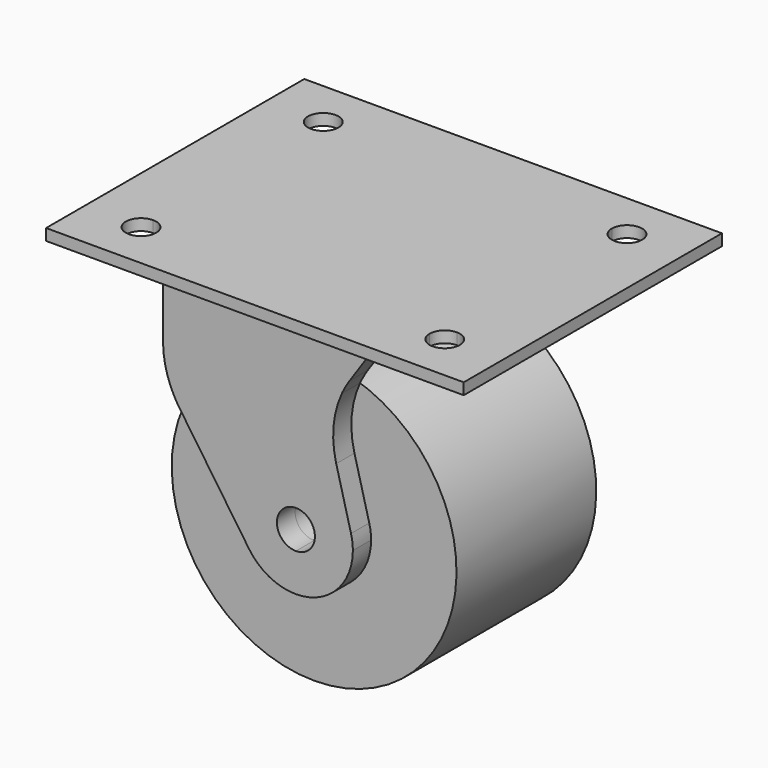
from build123d import *

# Parameters (mm, degrees)
F1_DEPTH = 23
F2_W     = 110
F2_H     = 85
F3_DEPTH = 3
F5_DEPTH = 6
F6_W     = 34.7799539885
F6_H     = 6
F7_DEPTH = 1
F8_DEPTH = 1


with BuildPart() as f1:
    # F0 (on Front) → F1 (new body, symmetric)
    with BuildSketch(Plane.XZ):
        with BuildLine():
            ThreePointArc((37.5, -57.5), (-26.5165042945, -30.9834957055), (0, -95))
            ThreePointArc((0, -95), (26.5165042945, -84.0165042945), (37.5, -57.5))
        make_face()
        with BuildLine():
            ThreePointArc((5, -57.5), (3.5355339059, -61.0355339059), (0, -62.5))
            ThreePointArc((0, -62.5), (-3.5355339059, -53.9644660941), (5, -57.5))
        make_face(mode=Mode.SUBTRACT)
    extrude(amount=F1_DEPTH, both=True)


with BuildPart() as f3:
    # F2 (on Top) → F3 (new body)
    with BuildSketch(Plane.XY):
        Rectangle(F2_W, F2_H)
        with BuildLine():
            Line((36, -30), (-36, -30))
            ThreePointArc((-36, -30), (-42.8284271247, -32.8284271247), (-40, -26))
            Line((-40, -26), (-40, 26))
            ThreePointArc((-40, 26), (-42.8284271247, 32.8284271247), (-36, 30))
            Line((-36, 30), (36, 30))
            ThreePointArc((36, 30), (40, 34), (44, 30))
            ThreePointArc((44, 30), (42.8284271247, 27.1715728753), (40, 26))
            Line((40, 26), (40, -26))
            ThreePointArc((40, -26), (42.8284271247, -27.1715728753), (44, -30))
            ThreePointArc((44, -30), (40, -34), (36, -30))
        make_face(mode=Mode.SUBTRACT)
        with BuildLine():
            ThreePointArc((-40, -26), (-37.1715728753, -27.1715728753), (-36, -30))
            Line((-36, -30), (36, -30))
            ThreePointArc((36, -30), (37.1715728753, -27.1715728753), (40, -26))
            Line((40, -26), (40, 26))
            ThreePointArc((40, 26), (37.1715728753, 27.1715728753), (36, 30))
            Line((36, 30), (-36, 30))
            ThreePointArc((-36, 30), (-37.1715728753, 27.1715728753), (-40, 26))
            Line((-40, 26), (-40, -26))
        make_face()
    extrude(amount=-F3_DEPTH)

    # F6 (on face) → F7 (cut)
    with BuildSketch(Plane(origin=(0, 0, -3), x_dir=(1, 0, 0), z_dir=(0, 0, -1))):
        Polygon((24.8050460115, -22.5), (0, -22.5), (0, -28.5), (24.8050460115, -28.6190058787), align=None)
        with Locations((-17.3899769943, -25.5)):
            Rectangle(F6_W, F6_H)
        Polygon((0, 22.5), (24.8050460115, 22.5), (24.8050460115, 28.6190058787), (0, 28.5), (-34.7799539885, 28.5), (-34.7799539885, 22.5), align=None)
    extrude(amount=-F7_DEPTH, mode=Mode.SUBTRACT)


with BuildPart() as f5:
    # F4 (on face) → F5 (new body)
    with BuildSketch(Plane.XZ.offset(23)):
        with BuildLine():
            ThreePointArc((-31.7587456306, -37.5592859714), (-12.5289492083, -22.1549093687), (12.1096103032, -22.0090527274))
            ThreePointArc((12.1096103032, -22.0090527274), (13.0382727302, -20.194540616), (14.1116697761, -18.4617143444))
            Line((14.1116697761, -18.4617143444), (24.5849639177, -3))
            Line((24.5849639177, -3), (0, -3))
            Line((0, -3), (-35, -3))
            Line((-35, -3), (-35, -25.248437561))
            ThreePointArc((-35, -25.248437561), (-34.1761105305, -31.6136303796), (-31.7587456306, -37.5592859714))
        make_face()
        with BuildLine():
            ThreePointArc((-12.3687979141, -65.9860378364), (-6.2301711882, -43.8550387701), (14.5137450016, -53.7117014336))
            Line((14.5137450016, -53.7117014336), (10.6205409153, -38.7960419739))
            ThreePointArc((10.6205409153, -38.7960419739), (9.9078937869, -30.273289816), (12.1096103032, -22.0090527274))
            ThreePointArc((12.1096103032, -22.0090527274), (-12.5289492083, -22.1549093687), (-31.7587456306, -37.5592859714))
            ThreePointArc((-31.7587456306, -37.5592859714), (-31.2065084773, -38.4879238879), (-30.6146631901, -39.3918339551))
            Line((-30.6146631901, -39.3918339551), (-12.3687979141, -65.9860378364))
        make_face()
        with BuildLine():
            ThreePointArc((-12.3687979141, -65.9860378364), (4.4422984641, -71.8271066289), (15, -57.5))
            ThreePointArc((15, -57.5), (14.8779396259, -55.5903108924), (14.5137450016, -53.7117014336))
            ThreePointArc((14.5137450016, -53.7117014336), (-6.2301711882, -43.8550387701), (-12.3687979141, -65.9860378364))
        make_face()
        with BuildLine():
            ThreePointArc((0, -62.5), (-3.5355339059, -53.9644660941), (5, -57.5))
            ThreePointArc((5, -57.5), (3.5355339059, -61.0355339059), (0, -62.5))
        make_face(mode=Mode.SUBTRACT)
    extrude(amount=F5_DEPTH)

    # F8 (add): a face of the model
    f8_faces = [f5.faces().sort_by_distance(p)[0] for p in [
        (-5.2075180411, -26, -3),
    ]]
    extrude(f8_faces, amount=F8_DEPTH)


solid = Compound([f1.part, f3.part, f5.part])
